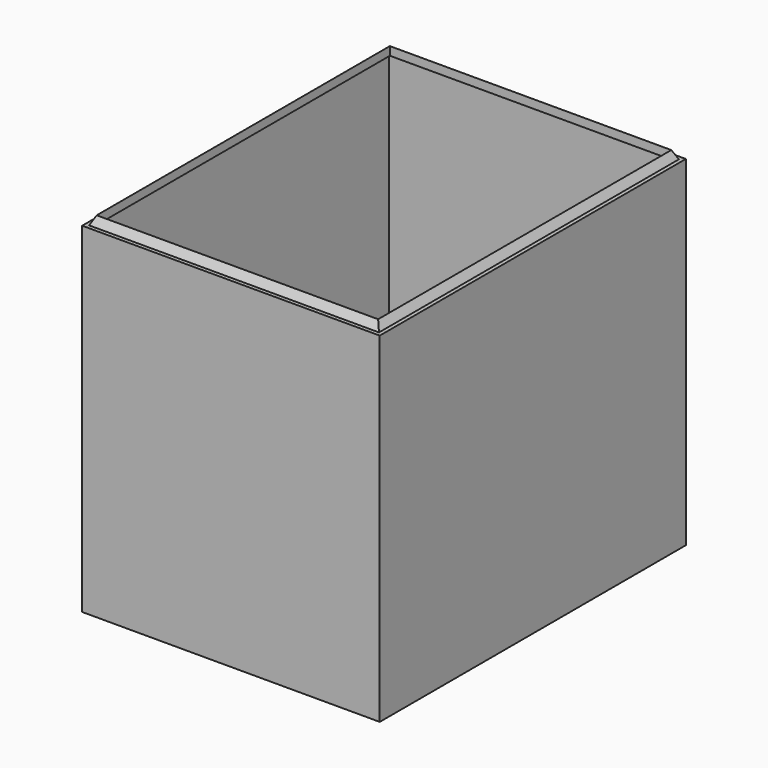
from build123d import *

# Parameters (mm, degrees)
F0_W     = 140
F0_H     = 180
F1_DEPTH = 160
F2_T     = -1.8
F3_W     = 136.4
F3_H     = 176.4
F5_W     = 132.4
F5_H     = 172.4
F8_DEPTH = 25


# Not quite as in the source:
# - the program builds the solid bodies; features that only make, move or delete a surface that nothing else refers to are left out


with BuildPart() as f1:
    # F0 (on Top) → F1 (new body)
    with BuildSketch(Plane.XY):
        Rectangle(F0_W, F0_H)
    extrude(amount=F1_DEPTH)

    # F2
    f2_openings = [f1.faces().sort_by_distance(p)[0] for p in [
        (0, 0, 160),
    ]]
    offset(amount=F2_T, openings=f2_openings)


with BuildPart() as f7:
    # F3 (on face) → F7 section 0
    with BuildSketch(Plane.XY.offset(160)):
        Rectangle(F3_W, F3_H)
    # F5 (on offset) → F7 section 1
    with BuildSketch(Plane.XY.offset(164)):
        Rectangle(F5_W, F5_H)
    loft()

    # F5 (on offset) → F8 (cut)
    with BuildSketch(Plane.XY.offset(164)):
        Rectangle(F5_W, F5_H)
    extrude(amount=-F8_DEPTH, mode=Mode.SUBTRACT)


solid = Compound([f1.part, f7.part])
